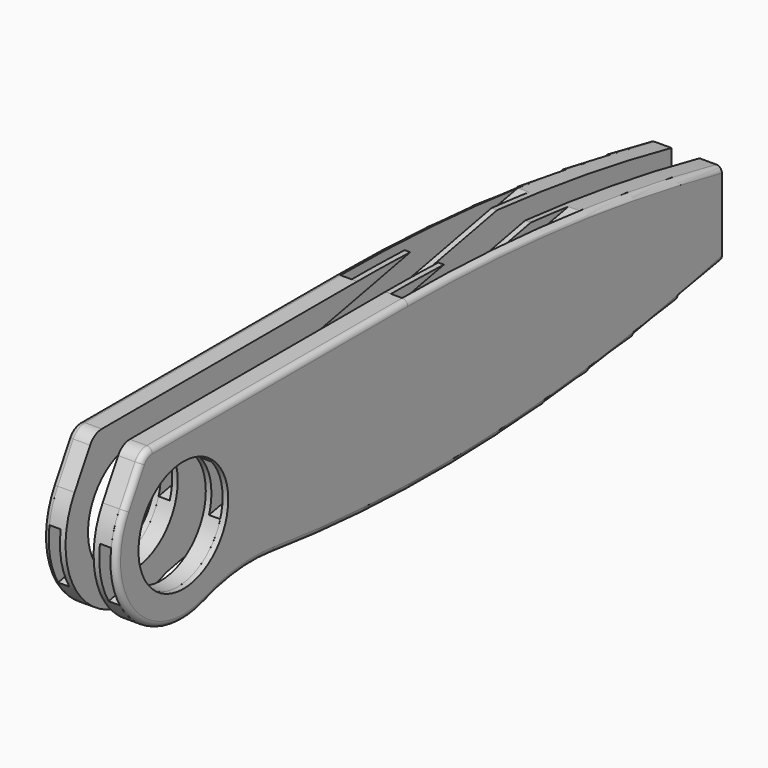
from build123d import *

# Parameters (mm, degrees)
F1_R     = 10
F2_DEPTH = 3
F4_DEPTH = 2
F6_DEPTH = 1.001
F7_START = 3
F7_DEPTH = 1
F8_R     = 0.99999


# Not quite as in the source:
# - a fillet or chamfer is up to 0.001 mm smaller than in the source, because OpenCascade refuses the exact size


with BuildPart() as f2:
    # F1 (on offset) → F2 (new body)
    with BuildSketch(Plane.YZ.offset(2.5)):
        with BuildLine():
            Line((-9.5262794416, 13.5), (-12.9903810568, 7.5))
            ThreePointArc((-12.9903810568, 7.5), (-11.5350360185, -9.5886883385), (5, -14.1421356237))
            ThreePointArc((5, -14.1421356237), (12.4075163283, -12.4727233008), (20, -12.5842013328))
            ThreePointArc((20, -12.5842013328), (70.2340902125, -14.6463678304), (120, -7.5))
            Line((120, -7.5), (120, 7.5))
            ThreePointArc((120, 7.5), (85.2003196008, 13.1196496077), (50, 15))
            Line((50, 15), (-6.9282032303, 15))
            ThreePointArc((-6.9282032303, 15), (-8.4282032303, 14.5980762114), (-9.5262794416, 13.5))
        make_face()
        Circle(F1_R, mode=Mode.SUBTRACT)
    extrude(amount=F2_DEPTH)

    # F3 (on face) → F4 (cut)
    with BuildSketch(Plane.YZ.offset(5.5)):
        Polygon((50, 15), (-25.7355715851, 0), (-25.7355715851, -10.1942473186), (101.4711431703, 15), align=None)
    extrude(amount=-F4_DEPTH, mode=Mode.SUBTRACT)

    # F5 (on face) → F6 (cut, through all)
    with BuildSketch(Plane.YZ.offset(3.5)):
        with BuildLine():
            Line((61.8030459338, 14.7891202569), (38.7521068975, 10.2237082806))
            ThreePointArc((38.7521068975, 10.2237082806), (36.7854524498, 7.2856357349), (39.7235249955, 5.3189812873))
            Line((39.7235249955, 5.3189812873), (87.538617519, 14.7891202569))
            Line((87.538617519, 14.7891202569), (61.8030459338, 14.7891202569))
        make_face()
    extrude(amount=-F6_DEPTH, mode=Mode.SUBTRACT)


with BuildPart() as f7:
    # F1 (on offset) → F7 (new body)
    with BuildSketch(Plane.YZ.offset(2.5).offset(F7_START)):
        with BuildLine():
            Line((-9.5262794416, 13.5), (-12.9903810568, 7.5))
            ThreePointArc((-12.9903810568, 7.5), (-11.5350360185, -9.5886883385), (5, -14.1421356237))
            ThreePointArc((5, -14.1421356237), (12.4075163283, -12.4727233008), (20, -12.5842013328))
            ThreePointArc((20, -12.5842013328), (70.2340902125, -14.6463678304), (120, -7.5))
            Line((120, -7.5), (120, 7.5))
            ThreePointArc((120, 7.5), (85.2003196008, 13.1196496077), (50, 15))
            Line((50, 15), (-6.9282032303, 15))
            ThreePointArc((-6.9282032303, 15), (-8.4282032303, 14.5980762114), (-9.5262794416, 13.5))
        make_face()
        Circle(F1_R, mode=Mode.SUBTRACT)
    extrude(amount=F7_DEPTH)

    # F8 (radius 1 in the source; OpenCascade refuses exactly that, so slightly less here)
    f8_edges = [f7.edges().sort_by_distance(p)[0] for p in [
        (6.5, -11.25833, 10.5),
    ]]
    fillet(f8_edges, radius=F8_R)


with BuildPart() as f9_1:
    # F9: instance of F2
    add(f2.part.mirror(Plane.YZ))


with BuildPart() as f9_2:
    # F9: instance of F7
    add(f7.part.mirror(Plane.YZ))


solid = Compound([f2.part, f7.part, f9_1.part, f9_2.part])
